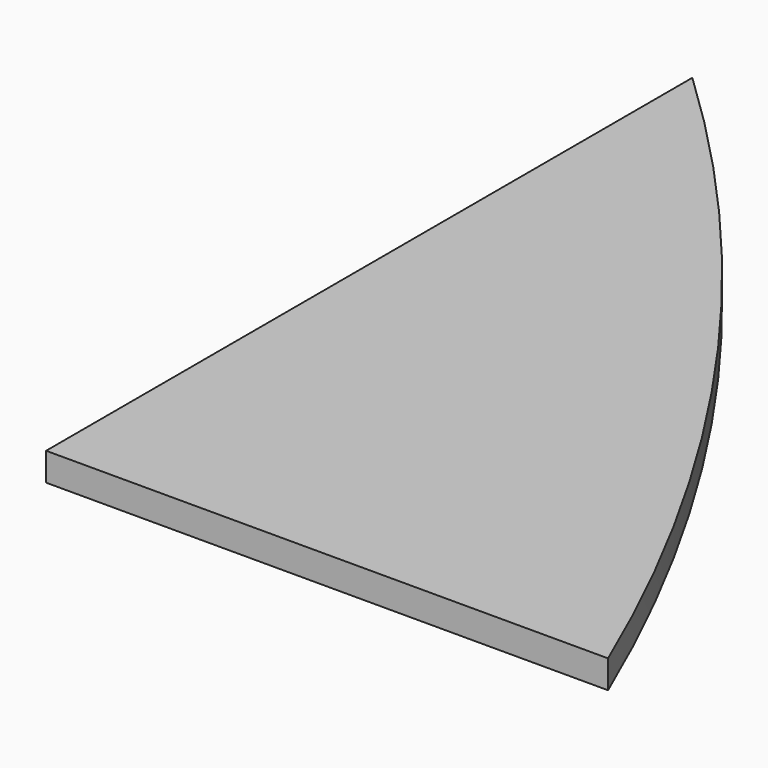
from build123d import *

# Parameters (mm, degrees)
F1_DEPTH = 4


# Not quite as in the source:
# - a feature names something its author has since deleted; it is built from what else it names


with BuildPart() as f1:
    # F0 (on Top) → F1 (new body)
    with BuildSketch(Plane.XY):
        with BuildLine():
            ThreePointArc((33.089133976, -73.1535100713), (-0.9595332134, -11.5134524639), (-46.910866024, 41.8464899287))
            Line((-46.910866024, 41.8464899287), (-46.910866024, -73.1535100713))
            Line((-46.910866024, -73.1535100713), (33.089133976, -73.1535100713))
        make_face()
    extrude(amount=F1_DEPTH)


solid = f1.part
